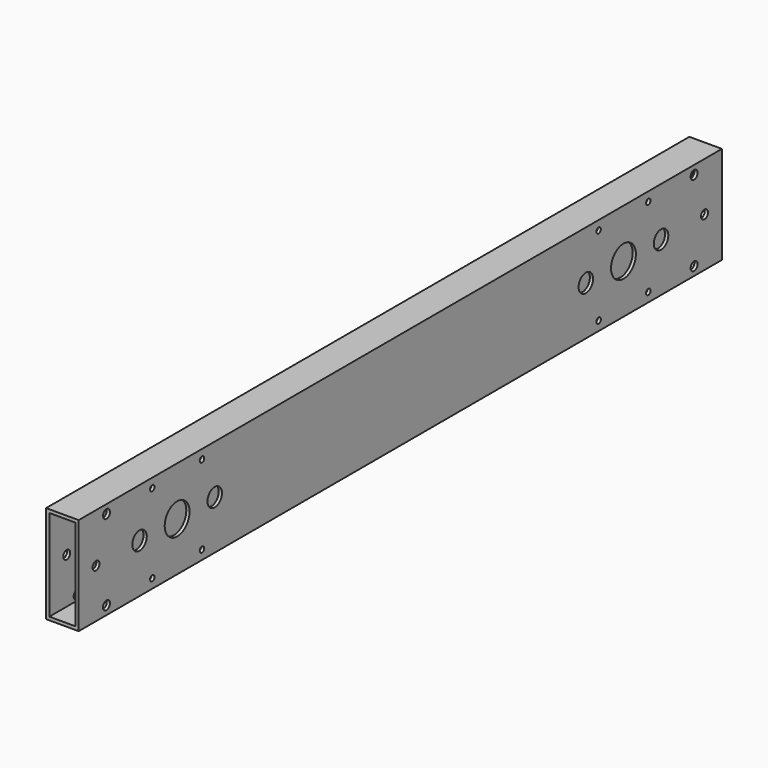
from build123d import *

# Parameters (mm, degrees)
F0_W     = 30
F0_H     = 90
F1_DEPTH = 370
F2_T     = -3
F3_R     = 2.5527
F3_R_2   = 14.28115
F3_R_3   = 8.3312
F4_DEPTH = 30.001
F5_R     = 4
F6_DEPTH = 30.001


# Not quite as in the source:
# - a pattern or mirror of a feature is missing from the dataset's text; its kind, count and spacing are read off the source's solid


with BuildPart() as f1:
    # F0 (on Front) → F1 (new body, symmetric)
    with BuildSketch(Plane.XZ):
        Rectangle(F0_W, F0_H)
    extrude(amount=F1_DEPTH, both=True)

    # F2
    f2_openings = [f1.faces().sort_by_distance(p)[0] for p in [
        (0, -370, 0),
        (0, 370, 0),
    ]]
    offset(amount=F2_T, openings=f2_openings)

    # F3 (on face) → F4 (cut, through all)
    with BuildSketch(Plane.YZ.offset(15)):
        with Locations((228.1688, 36.5125)):
            Circle(F3_R)
        with Locations((228.1688, -36.5125)):
            Circle(F3_R)
        with Locations((285.3188, -36.5125)):
            Circle(F3_R)
        with Locations((285.3188, 36.5125)):
            Circle(F3_R)
        with Locations((256.7438, 0)):
            Circle(F3_R_2)
        with Locations((213.4876, 0)):
            Circle(F3_R_3)
        with Locations((300, 0)):
            Circle(F3_R_3)
    f4 = extrude(amount=-F4_DEPTH, mode=Mode.SUBTRACT)

    # F4_copies: F4 across plane
    add(f4.mirror(Plane(origin=(0, 0, 0), x_dir=(0, 0, -1), z_dir=(0, -1, 0))), mode=Mode.SUBTRACT)

    # F5 (on face) → F6 (cut, through all)
    with BuildSketch(Plane.YZ.offset(15)):
        with Locations((-338, 37)):
            Circle(F5_R)
        with Locations((-350, 0)):
            Circle(F5_R)
        with Locations((-338, -37)):
            Circle(F5_R)
    f6 = extrude(amount=-F6_DEPTH, mode=Mode.SUBTRACT)

    # F6_copies: F6 across plane
    add(f6.mirror(Plane.ZX), mode=Mode.SUBTRACT)


solid = f1.part
